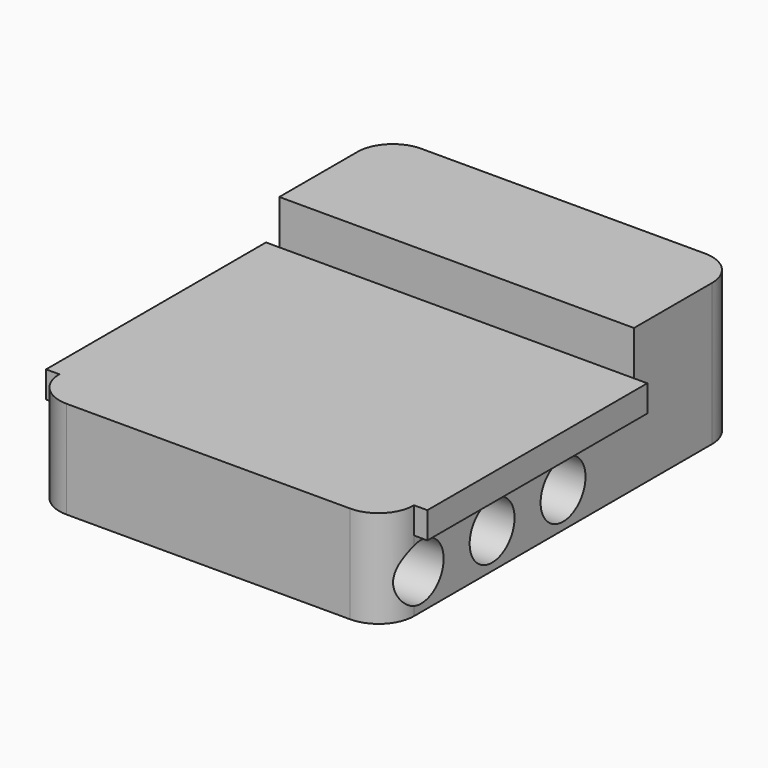
from build123d import *

# Parameters (mm, degrees)
F0_W         = 50.8
F0_H         = 38.1
F1_DEPTH     = 10.16
F2_R         = 4.01955
F3_DEPTH     = 23.495
F4_R         = 4.01955
F5_DEPTH     = 23.495
F6_DEPTH     = 25.4
F7_W         = 50.8
F7_H         = 19.05
F8_DEPTH     = 10.16
F9_R         = 4.01955
F10_DEPTH    = 15.24
F11_T1_DEPTH = 35.56
F12_T1_DEPTH = 45.72
F13_DEPTH    = 3.81
F15_W        = 39.37
F15_H        = 3.81
F16_DEPTH    = 1.905
F14_W        = 39.37
F14_H        = 3.81
F17_DEPTH    = 1.905


# Not quite as in the source:
# - a fillet or chamfer that OpenCascade refuses, or shapes differently, is made with other operations: its cross-section is extruded or revolved along the edge and cut away or added


with BuildPart() as f1:
    # F0 (on Top) → F1 (new body)
    with BuildSketch(Plane.XY):
        Rectangle(F0_W, F0_H)
    extrude(amount=F1_DEPTH)

    # F2 (on face) → F3 (cut)
    with BuildSketch(Plane(origin=(-25.4, 0, 0), x_dir=(0, -1, 0), z_dir=(-1, 0, 0))):
        with Locations((-12.7, 5.08)):
            Circle(F2_R)
        with Locations((0, 5.08)):
            Circle(F2_R)
        with Locations((12.7, 5.08)):
            Circle(F2_R)
    extrude(amount=-F3_DEPTH, mode=Mode.SUBTRACT)

    # F4 (on face) → F5 (cut)
    with BuildSketch(Plane.YZ.offset(25.4)):
        with Locations((-12.7, 5.08)):
            Circle(F4_R)
        with Locations((0, 5.08)):
            Circle(F4_R)
        with Locations((12.7, 5.08)):
            Circle(F4_R)
    extrude(amount=-F5_DEPTH, mode=Mode.SUBTRACT)

    # F6 (add): a face of the model
    f6_faces = [f1.faces().sort_by_distance(p)[0] for p in [
        (0, 19.05, 5.08),
    ]]
    extrude(f6_faces, amount=F6_DEPTH)

    # F7 (on face) → F8 (join)
    with BuildSketch(Plane.XY.offset(10.16)):
        with Locations((0, 34.925)):
            Rectangle(F7_W, F7_H)
    extrude(amount=F8_DEPTH)

    # F9 (on face) → F10 (cut)
    with BuildSketch(Plane(origin=(0, 44.45, 0), x_dir=(-1, 0, 0), z_dir=(0, 1, 0))):
        with Locations((0, 5.08)):
            Circle(F9_R)
        with Locations((-8.001, 15.24)):
            Circle(F9_R)
        with Locations((-18.84045, 5.08)):
            Circle(F9_R)
        with Locations((8.001, 15.24)):
            Circle(F9_R)
        with Locations((18.84045, 5.08)):
            Circle(F9_R)
    extrude(amount=-F10_DEPTH, mode=Mode.SUBTRACT)

    # F11: fillet of radius 5.08 on 2 edges, made by hand

    # F11_s2 → F11_t1 (cut)
    with BuildSketch(Plane.XY.offset(-12.7)):
        with BuildLine():
            ThreePointArc((-20.32, -19.05), (-23.9121024484, -17.5621024484), (-25.4, -13.97))
            Line((-25.4, -13.97), (-25.4, -19.05))
            Line((-25.4, -19.05), (-20.32, -19.05))
        make_face()
        with BuildLine():
            ThreePointArc((20.32, -19.05), (23.9121024484, -17.5621024484), (25.4, -13.97))
            Line((25.4, -13.97), (25.4, -19.05))
            Line((25.4, -19.05), (20.32, -19.05))
        make_face()
    extrude(amount=F11_T1_DEPTH, mode=Mode.SUBTRACT)

    # F12: fillet of radius 5.08 on 2 edges, made by hand

    # F12_s2 → F12_t1 (cut)
    with BuildSketch(Plane.XY.offset(-12.7)):
        with BuildLine():
            ThreePointArc((-25.4, 39.37), (-23.9121024484, 42.9621024484), (-20.32, 44.45))
            Line((-20.32, 44.45), (-25.4, 44.45))
            Line((-25.4, 44.45), (-25.4, 39.37))
        make_face()
        with BuildLine():
            ThreePointArc((20.32, 44.45), (23.9121024484, 42.9621024484), (25.4, 39.37))
            Line((25.4, 39.37), (25.4, 44.45))
            Line((25.4, 44.45), (20.32, 44.45))
        make_face()
    extrude(amount=F12_T1_DEPTH, mode=Mode.SUBTRACT)

    # F13 (add): a face of the model
    f13_faces = [f1.faces().sort_by_distance(p)[0] for p in [
        (0, 3.2789617265, 10.16),
    ]]
    extrude(f13_faces, amount=F13_DEPTH)

    # F15 (on face) → F16 (join)
    with BuildSketch(Plane(origin=(-25.4, 0, 0), x_dir=(0, -1, 0), z_dir=(-1, 0, 0))):
        with Locations((-5.715, 12.065)):
            Rectangle(F15_W, F15_H)
    extrude(amount=F16_DEPTH)

    # F14 (on face) → F17 (join)
    with BuildSketch(Plane.YZ.offset(25.4)):
        with Locations((5.715, 12.065)):
            Rectangle(F14_W, F14_H)
    extrude(amount=F17_DEPTH)


solid = f1.part
